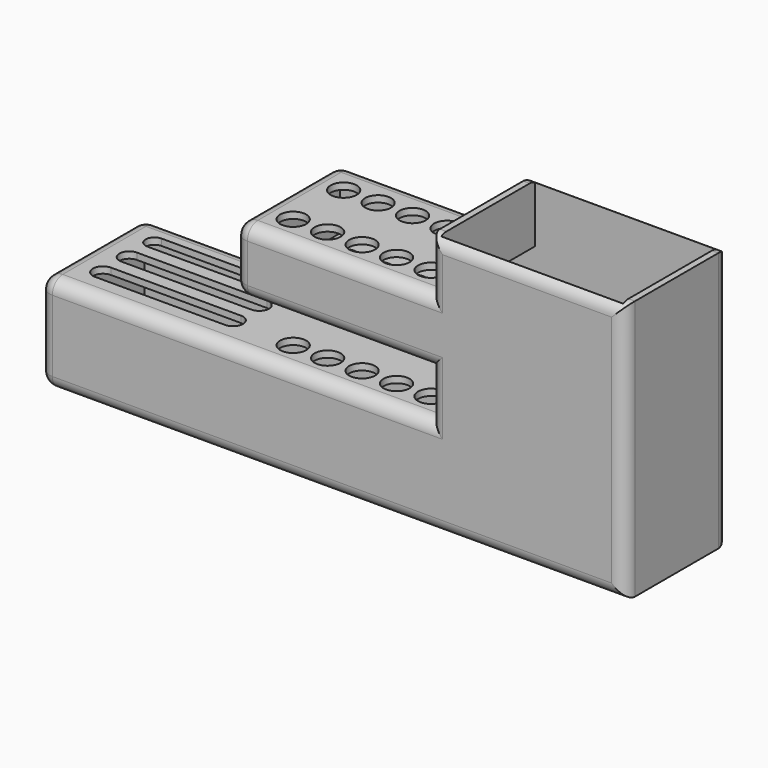
from build123d import *

# Parameters (mm, degrees)
F0_W          = 76.2
F0_H          = 25.4
F0_W_2        = 152.4
F0_H_2        = 38.1
F1_DEPTH      = 50.8
F2_T          = -2.54
F3_R          = 5.08
F4_DEPTH      = 76.2
F5_T1_DEPTH   = 101.6
F5_T3_DEPTH   = 32.8448284238
F5_T5_DEPTH   = 71.12
F5_T7_DEPTH   = 15.24
F5_T9_DEPTH   = 17.9551715762
F5_T11_DEPTH  = 147.32
F5_T13_DEPTH  = 27.94
F5_T15_DEPTH  = 236.22
F5_T17_DEPTH  = 127
F5_T19_DEPTH  = 40.64
F5_S23_W      = 5.08
F5_S23_H      = 5.08
F5_T24_DEPTH  = 5.08
F5_S29_W      = 5.08
F5_S29_H      = 5.08
F5_T30_DEPTH  = 5.08
F5_S35_W      = 5.08
F5_S35_H      = 5.08
F5_T36_DEPTH  = 5.08
F5_S41_W      = 5.08
F5_S41_H      = 5.08
F5_T42_DEPTH  = 5.08
F5_S47_W      = 5.08
F5_S47_H      = 5.08
F5_T48_DEPTH  = 5.08
F5_S53_W      = 5.08
F5_S53_H      = 5.08
F5_T54_DEPTH  = 5.08
F5_S59_W      = 5.08
F5_S59_H      = 5.08
F5_T60_DEPTH  = 5.08
F5_S65_W      = 5.08
F5_S65_H      = 5.08
F5_T66_DEPTH  = 5.08
F5_T73_DEPTH  = 45.5448284238
F5_T77_DEPTH  = 83.82
F5_T84_DEPTH  = 83.82
F5_T88_DEPTH  = 30.6551715762
F5_T95_DEPTH  = 30.6551715762
F5_T99_DEPTH  = 160.02
F5_T106_DEPTH = 45.5448284238
F5_T110_DEPTH = 83.82
F5_T117_DEPTH = 83.82
F5_T121_DEPTH = 30.6551715762
F5_T128_DEPTH = 30.6551715762
F5_T132_DEPTH = 160.02
F7_DEPTH      = 25.4


# Not quite as in the source:
# - a fillet or chamfer that OpenCascade refuses, or shapes differently, is made with other operations: its cross-section is extruded or revolved along the edge and cut away or added


with BuildPart() as f1:
    # F0 (on Front) → F1 (new body)
    with BuildSketch(Plane.XZ):
        Polygon((76.2, 45.5448284238), (0, 45.5448284238), (0, 25.4), (0, 0), (0, -17.9551715762), (0, -56.0551715762), (76.2, -56.0551715762), align=None)
        with Locations((-38.1, 12.7)):
            Rectangle(F0_W, F0_H)
        with Locations((-76.2, -37.0051715762)):
            Rectangle(F0_W_2, F0_H_2)
    extrude(amount=-F1_DEPTH)

    # F2
    f2_openings = [f1.faces().sort_by_distance(p)[0] for p in [
        (38.1, 25.4, 45.544828),
    ]]
    offset(amount=F2_T, openings=f2_openings, kind=Kind.INTERSECTION)

    # F3 (on face) → F4 (cut)
    with BuildSketch(Plane.XY.offset(25.4)):
        with Locations((-9.3213441366, 12.3962962994)):
            Circle(F3_R)
        with Locations((-9.3213441366, 37.0342962994)):
            Circle(F3_R)
        with Locations((-22.7833441366, 12.3962962994)):
            Circle(F3_R)
        with Locations((-22.7833441366, 37.0342962994)):
            Circle(F3_R)
        with Locations((-36.2453441366, 12.3962962994)):
            Circle(F3_R)
        with Locations((-36.2453441366, 37.0342962994)):
            Circle(F3_R)
        with Locations((-49.7073441366, 12.3962962994)):
            Circle(F3_R)
        with Locations((-49.7073441366, 37.0342962994)):
            Circle(F3_R)
        with Locations((-63.1693441366, 12.3962962994)):
            Circle(F3_R)
        with Locations((-63.1693441366, 37.0342962994)):
            Circle(F3_R)
    extrude(amount=-F4_DEPTH, mode=Mode.SUBTRACT)

    # F5: fillet of radius 5.08 on 24 edges, made by hand

    # F5_s2 → F5_t1 (cut)
    with BuildSketch(Plane.YZ.offset(-12.7)):
        with BuildLine():
            ThreePointArc((5.08, 45.5448284238), (1.4878975516, 44.0569308722), (0, 40.4648284238))
            Line((0, 40.4648284238), (0, 45.5448284238))
            Line((0, 45.5448284238), (5.08, 45.5448284238))
        make_face()
        with BuildLine():
            ThreePointArc((45.72, 45.5448284238), (49.3121024484, 44.0569308722), (50.8, 40.4648284238))
            Line((50.8, 40.4648284238), (50.8, 45.5448284238))
            Line((50.8, 45.5448284238), (45.72, 45.5448284238))
        make_face()
    extrude(amount=F5_T1_DEPTH, mode=Mode.SUBTRACT)

    # F5_s4 → F5_t3 (cut)
    with BuildSketch(Plane.XY.offset(25.4)):
        with BuildLine():
            ThreePointArc((0, 5.08), (1.4878975516, 1.4878975516), (5.08, 0))
            Line((5.08, 0), (0, 0))
            Line((0, 0), (0, 5.08))
        make_face()
        with BuildLine():
            ThreePointArc((0, 45.72), (1.4878975516, 49.3121024484), (5.08, 50.8))
            Line((5.08, 50.8), (0, 50.8))
            Line((0, 50.8), (0, 45.72))
        make_face()
    extrude(amount=F5_T3_DEPTH, mode=Mode.SUBTRACT)

    # F5_s6 → F5_t5 (cut)
    with BuildSketch(Plane.YZ.offset(-71.12)):
        with BuildLine():
            ThreePointArc((5.08, 25.4), (1.4878975516, 23.9121024484), (0, 20.32))
            Line((0, 20.32), (0, 25.4))
            Line((0, 25.4), (5.08, 25.4))
        make_face()
        with BuildLine():
            ThreePointArc((0, 5.08), (1.4878975516, 1.4878975516), (5.08, 0))
            Line((5.08, 0), (0, 0))
            Line((0, 0), (0, 5.08))
        make_face()
        with BuildLine():
            ThreePointArc((45.72, 25.4), (49.3121024484, 23.9121024484), (50.8, 20.32))
            Line((50.8, 20.32), (50.8, 25.4))
            Line((50.8, 25.4), (45.72, 25.4))
        make_face()
        with BuildLine():
            ThreePointArc((50.8, 5.08), (49.3121024484, 1.4878975516), (45.72, 0))
            Line((45.72, 0), (50.8, 0))
            Line((50.8, 0), (50.8, 5.08))
        make_face()
    extrude(amount=F5_T5_DEPTH, mode=Mode.SUBTRACT)

    # F5_s8 → F5_t7 (cut)
    with BuildSketch(Plane.XY.offset(5.08)):
        with BuildLine():
            ThreePointArc((-71.12, 0), (-74.7121024484, 1.4878975516), (-76.2, 5.08))
            Line((-76.2, 5.08), (-76.2, 0))
            Line((-76.2, 0), (-71.12, 0))
        make_face()
        with BuildLine():
            ThreePointArc((-71.12, 50.8), (-74.7121024484, 49.3121024484), (-76.2, 45.72))
            Line((-76.2, 45.72), (-76.2, 50.8))
            Line((-76.2, 50.8), (-71.12, 50.8))
        make_face()
    extrude(amount=F5_T7_DEPTH, mode=Mode.SUBTRACT)

    # F5_s10 → F5_t9 (cut)
    with BuildSketch(Plane.XY.offset(-17.9551715762)):
        with BuildLine():
            ThreePointArc((5.08, 0), (1.4878975516, 1.4878975516), (0, 5.08))
            Line((0, 5.08), (0, 0))
            Line((0, 0), (5.08, 0))
        make_face()
        with BuildLine():
            ThreePointArc((5.08, 50.8), (1.4878975516, 49.3121024484), (0, 45.72))
            Line((0, 45.72), (0, 50.8))
            Line((0, 50.8), (5.08, 50.8))
        make_face()
    extrude(amount=F5_T9_DEPTH, mode=Mode.SUBTRACT)

    # F5_s12 → F5_t11 (cut)
    with BuildSketch(Plane.YZ.offset(-147.32)):
        with BuildLine():
            ThreePointArc((0, -23.0351715762), (1.4878975516, -19.4430691278), (5.08, -17.9551715762))
            Line((5.08, -17.9551715762), (0, -17.9551715762))
            Line((0, -17.9551715762), (0, -23.0351715762))
        make_face()
        with BuildLine():
            ThreePointArc((50.8, -23.0351715762), (49.3121024484, -19.4430691278), (45.72, -17.9551715762))
            Line((45.72, -17.9551715762), (50.8, -17.9551715762))
            Line((50.8, -17.9551715762), (50.8, -23.0351715762))
        make_face()
    extrude(amount=F5_T11_DEPTH, mode=Mode.SUBTRACT)

    # F5_s14 → F5_t13 (cut)
    with BuildSketch(Plane.XY.offset(-50.9751715762)):
        with BuildLine():
            ThreePointArc((-147.32, 0), (-150.9121024484, 1.4878975516), (-152.4, 5.08))
            Line((-152.4, 5.08), (-152.4, 0))
            Line((-152.4, 0), (-147.32, 0))
        make_face()
        with BuildLine():
            ThreePointArc((-147.32, 50.8), (-150.9121024484, 49.3121024484), (-152.4, 45.72))
            Line((-152.4, 45.72), (-152.4, 50.8))
            Line((-152.4, 50.8), (-147.32, 50.8))
        make_face()
    extrude(amount=F5_T13_DEPTH, mode=Mode.SUBTRACT)

    # F5_s16 → F5_t15 (cut)
    with BuildSketch(Plane.YZ.offset(-147.32)):
        with BuildLine():
            ThreePointArc((0, -50.9751715762), (1.4878975516, -54.5672740246), (5.08, -56.0551715762))
            Line((5.08, -56.0551715762), (0, -56.0551715762))
            Line((0, -56.0551715762), (0, -50.9751715762))
        make_face()
        with BuildLine():
            ThreePointArc((50.8, -50.9751715762), (49.3121024484, -54.5672740246), (45.72, -56.0551715762))
            Line((45.72, -56.0551715762), (50.8, -56.0551715762))
            Line((50.8, -56.0551715762), (50.8, -50.9751715762))
        make_face()
    extrude(amount=F5_T15_DEPTH, mode=Mode.SUBTRACT)

    # F5_s18 → F5_t17 (cut)
    with BuildSketch(Plane.XY.offset(-68.7551715762)):
        with BuildLine():
            ThreePointArc((71.12, 0), (74.7121024484, 1.4878975516), (76.2, 5.08))
            Line((76.2, 5.08), (76.2, 0))
            Line((76.2, 0), (71.12, 0))
        make_face()
        with BuildLine():
            ThreePointArc((71.12, 50.8), (74.7121024484, 49.3121024484), (76.2, 45.72))
            Line((76.2, 45.72), (76.2, 50.8))
            Line((76.2, 50.8), (71.12, 50.8))
        make_face()
    extrude(amount=F5_T17_DEPTH, mode=Mode.SUBTRACT)

    # F5_s20 → F5_t19 (cut)
    with BuildSketch(Plane.XZ.offset(-45.72)):
        with BuildLine():
            ThreePointArc((-147.32, -17.9551715762), (-150.9121024484, -19.4430691278), (-152.4, -23.0351715762))
            Line((-152.4, -23.0351715762), (-152.4, -17.9551715762))
            Line((-152.4, -17.9551715762), (-147.32, -17.9551715762))
        make_face()
        with BuildLine():
            ThreePointArc((-152.4, -50.9751715762), (-150.9121024484, -54.5672740246), (-147.32, -56.0551715762))
            Line((-147.32, -56.0551715762), (-152.4, -56.0551715762))
            Line((-152.4, -56.0551715762), (-152.4, -50.9751715762))
        make_face()
        with BuildLine():
            ThreePointArc((-71.12, 25.4), (-74.7121024484, 23.9121024484), (-76.2, 20.32))
            Line((-76.2, 20.32), (-76.2, 25.4))
            Line((-76.2, 25.4), (-71.12, 25.4))
        make_face()
        with BuildLine():
            ThreePointArc((-76.2, 5.08), (-74.7121024484, 1.4878975516), (-71.12, 0))
            Line((-71.12, 0), (-76.2, 0))
            Line((-76.2, 0), (-76.2, 5.08))
        make_face()
    extrude(amount=F5_T19_DEPTH, mode=Mode.SUBTRACT)


with BuildPart() as f5_tool22:
    # F5_s23 → F5_t24 (new body)
    with BuildSketch(Plane.YZ.offset(-71.12)):
        with Locations((2.54, 22.86)):
            Rectangle(F5_S23_W, F5_S23_H)
    extrude(amount=-F5_T24_DEPTH)

    # F5_s25 → F5_t26 (revolve, cut)
    with BuildSketch(Plane(origin=(-71.12, 5.08, 20.32), x_dir=(0, 0.7071067812, -0.7071067812), z_dir=(0, 0.7071067812, 0.7071067812))):
        with BuildLine():
            ThreePointArc((0, -5.08), (5.08, 0), (0, 5.08))
            Line((0, 5.08), (0, -5.08))
        make_face()
    revolve(axis=Axis((-71.12, 5.08, 20.32), (-1, 0, 0)), mode=Mode.SUBTRACT)


with BuildPart() as f1_1:
    add(f1.part)

    # F5_t21: cut F5_tool22
    add(f5_tool22.part, mode=Mode.SUBTRACT)


with BuildPart() as f5_tool28:
    # F5_s29 → F5_t30 (new body)
    with BuildSketch(Plane.YZ.offset(-71.12)):
        with Locations((2.54, 2.54)):
            Rectangle(F5_S29_W, F5_S29_H)
    extrude(amount=-F5_T30_DEPTH)

    # F5_s31 → F5_t32 (revolve, cut)
    with BuildSketch(Plane(origin=(-71.12, 5.08, 5.08), x_dir=(0, 0.7071067812, 0.7071067812), z_dir=(0, -0.7071067812, 0.7071067812))):
        with BuildLine():
            ThreePointArc((0, -5.08), (5.08, 0), (0, 5.08))
            Line((0, 5.08), (0, -5.08))
        make_face()
    revolve(axis=Axis((-71.12, 5.08, 5.08), (-1, 0, 0)), mode=Mode.SUBTRACT)


with BuildPart() as f1_2:
    add(f1_1.part)

    # F5_t27: cut F5_tool28
    add(f5_tool28.part, mode=Mode.SUBTRACT)


with BuildPart() as f5_tool34:
    # F5_s35 → F5_t36 (new body)
    with BuildSketch(Plane.YZ.offset(-147.32)):
        with Locations((2.54, -20.4951715762)):
            Rectangle(F5_S35_W, F5_S35_H)
    extrude(amount=-F5_T36_DEPTH)

    # F5_s37 → F5_t38 (revolve, cut)
    with BuildSketch(Plane(origin=(-147.32, 5.08, -23.0351715762), x_dir=(0, 0.7071067812, -0.7071067812), z_dir=(0, 0.7071067812, 0.7071067812))):
        with BuildLine():
            ThreePointArc((0, -5.08), (5.08, 0), (0, 5.08))
            Line((0, 5.08), (0, -5.08))
        make_face()
    revolve(axis=Axis((-147.32, 5.08, -23.0351715762), (-1, 0, 0)), mode=Mode.SUBTRACT)


with BuildPart() as f1_3:
    add(f1_2.part)

    # F5_t33: cut F5_tool34
    add(f5_tool34.part, mode=Mode.SUBTRACT)


with BuildPart() as f5_tool40:
    # F5_s41 → F5_t42 (new body)
    with BuildSketch(Plane.YZ.offset(-147.32)):
        with Locations((2.54, -53.5151715762)):
            Rectangle(F5_S41_W, F5_S41_H)
    extrude(amount=-F5_T42_DEPTH)

    # F5_s43 → F5_t44 (revolve, cut)
    with BuildSketch(Plane(origin=(-147.32, 5.08, -50.9751715762), x_dir=(0, 0.7071067812, 0.7071067812), z_dir=(0, -0.7071067812, 0.7071067812))):
        with BuildLine():
            ThreePointArc((0, -5.08), (5.08, 0), (0, 5.08))
            Line((0, 5.08), (0, -5.08))
        make_face()
    revolve(axis=Axis((-147.32, 5.08, -50.9751715762), (-1, 0, 0)), mode=Mode.SUBTRACT)


with BuildPart() as f1_4:
    add(f1_3.part)

    # F5_t39: cut F5_tool40
    add(f5_tool40.part, mode=Mode.SUBTRACT)


with BuildPart() as f5_tool46:
    # F5_s47 → F5_t48 (new body)
    with BuildSketch(Plane.XY.offset(20.32)):
        with Locations((-73.66, 48.26)):
            Rectangle(F5_S47_W, F5_S47_H)
    extrude(amount=F5_T48_DEPTH)

    # F5_s49 → F5_t50 (revolve, cut)
    with BuildSketch(Plane(origin=(-71.12, 45.72, 20.32), x_dir=(0.7071067812, -0.7071067812, 0), z_dir=(-0.7071067812, -0.7071067812, 0))):
        with BuildLine():
            ThreePointArc((0, -5.08), (5.08, 0), (0, 5.08))
            Line((0, 5.08), (0, -5.08))
        make_face()
    revolve(axis=Axis((-71.12, 45.72, 20.32), (0, 0, 1)), mode=Mode.SUBTRACT)


with BuildPart() as f1_5:
    add(f1_4.part)

    # F5_t45: cut F5_tool46
    add(f5_tool46.part, mode=Mode.SUBTRACT)


with BuildPart() as f5_tool52:
    # F5_s53 → F5_t54 (new body)
    with BuildSketch(Plane.YZ.offset(-71.12)):
        with Locations((48.26, 2.54)):
            Rectangle(F5_S53_W, F5_S53_H)
    extrude(amount=-F5_T54_DEPTH)

    # F5_s55 → F5_t56 (revolve, cut)
    with BuildSketch(Plane(origin=(-71.12, 45.72, 5.08), x_dir=(0, -0.7071067812, 0.7071067812), z_dir=(0, -0.7071067812, -0.7071067812))):
        with BuildLine():
            ThreePointArc((0, -5.08), (5.08, 0), (0, 5.08))
            Line((0, 5.08), (0, -5.08))
        make_face()
    revolve(axis=Axis((-71.12, 45.72, 5.08), (-1, 0, 0)), mode=Mode.SUBTRACT)


with BuildPart() as f1_6:
    add(f1_5.part)

    # F5_t51: cut F5_tool52
    add(f5_tool52.part, mode=Mode.SUBTRACT)


with BuildPart() as f5_tool58:
    # F5_s59 → F5_t60 (new body)
    with BuildSketch(Plane.YZ.offset(-147.32)):
        with Locations((48.26, -20.4951715762)):
            Rectangle(F5_S59_W, F5_S59_H)
    extrude(amount=-F5_T60_DEPTH)

    # F5_s61 → F5_t62 (revolve, cut)
    with BuildSketch(Plane(origin=(-147.32, 45.72, -23.0351715762), x_dir=(0, -0.7071067812, -0.7071067812), z_dir=(0, 0.7071067812, -0.7071067812))):
        with BuildLine():
            ThreePointArc((0, -5.08), (5.08, 0), (0, 5.08))
            Line((0, 5.08), (0, -5.08))
        make_face()
    revolve(axis=Axis((-147.32, 45.72, -23.0351715762), (-1, 0, 0)), mode=Mode.SUBTRACT)


with BuildPart() as f1_7:
    add(f1_6.part)

    # F5_t57: cut F5_tool58
    add(f5_tool58.part, mode=Mode.SUBTRACT)


with BuildPart() as f5_tool64:
    # F5_s65 → F5_t66 (new body)
    with BuildSketch(Plane.YZ.offset(-147.32)):
        with Locations((48.26, -53.5151715762)):
            Rectangle(F5_S65_W, F5_S65_H)
    extrude(amount=-F5_T66_DEPTH)

    # F5_s67 → F5_t68 (revolve, cut)
    with BuildSketch(Plane(origin=(-147.32, 45.72, -50.9751715762), x_dir=(0, -0.7071067812, 0.7071067812), z_dir=(0, -0.7071067812, -0.7071067812))):
        with BuildLine():
            ThreePointArc((0, -5.08), (5.08, 0), (0, 5.08))
            Line((0, 5.08), (0, -5.08))
        make_face()
    revolve(axis=Axis((-147.32, 45.72, -50.9751715762), (-1, 0, 0)), mode=Mode.SUBTRACT)


with BuildPart() as f1_8:
    add(f1_7.part)

    # F5_t63: cut F5_tool64
    add(f5_tool64.part, mode=Mode.SUBTRACT)


with BuildPart() as f5_tool71:
    # F5_s72 → F5_t73 (new body)
    with BuildSketch(Plane.XY.offset(58.2448284238)):
        with BuildLine():
            ThreePointArc((0, 5.08), (1.4878975516, 1.4878975516), (5.08, 0))
            Line((5.08, 0), (0, 0))
            Line((0, 0), (0, 5.08))
        make_face()
    extrude(amount=-F5_T73_DEPTH)

    split(bisect_by=Plane.XY.offset(25.4), keep=Keep.BOTTOM)


with BuildPart() as f5_tool75:
    # F5_s76 → F5_t77 (new body)
    with BuildSketch(Plane.YZ.offset(12.7)):
        with BuildLine():
            ThreePointArc((5.08, 25.4), (1.4878975516, 23.9121024484), (0, 20.32))
            Line((0, 20.32), (0, 25.4))
            Line((0, 25.4), (5.08, 25.4))
        make_face()
    extrude(amount=-F5_T77_DEPTH)

    split(bisect_by=Plane.YZ, keep=Keep.TOP)


with BuildPart() as f5_tool71_1:
    add(f5_tool71.part)

    # F5_t79: intersect F5_tool75
    add(f5_tool75.part, mode=Mode.INTERSECT)


with BuildPart() as f1_9:
    add(f1_8.part)

    # F5_t69: cut F5_tool71
    add(f5_tool71_1.part, mode=Mode.SUBTRACT)


with BuildPart() as f5_tool82:
    # F5_s83 → F5_t84 (new body)
    with BuildSketch(Plane.YZ.offset(-71.12)):
        with BuildLine():
            ThreePointArc((0, 5.08), (1.4878975516, 1.4878975516), (5.08, 0))
            Line((5.08, 0), (0, 0))
            Line((0, 0), (0, 5.08))
        make_face()
    extrude(amount=F5_T84_DEPTH)

    split(bisect_by=Plane.YZ, keep=Keep.TOP)


with BuildPart() as f5_tool86:
    # F5_s87 → F5_t88 (new body)
    with BuildSketch(Plane.XY.offset(12.7)):
        with BuildLine():
            ThreePointArc((5.08, 0), (1.4878975516, 1.4878975516), (0, 5.08))
            Line((0, 5.08), (0, 0))
            Line((0, 0), (5.08, 0))
        make_face()
    extrude(amount=-F5_T88_DEPTH)

    split(bisect_by=Plane.XY, keep=Keep.TOP)


with BuildPart() as f5_tool82_1:
    add(f5_tool82.part)

    # F5_t90: intersect F5_tool86
    add(f5_tool86.part, mode=Mode.INTERSECT)


with BuildPart() as f1_10:
    add(f1_9.part)

    # F5_t80: cut F5_tool82
    add(f5_tool82_1.part, mode=Mode.SUBTRACT)


with BuildPart() as f5_tool93:
    # F5_s94 → F5_t95 (new body)
    with BuildSketch(Plane.XY):
        with BuildLine():
            ThreePointArc((5.08, 0), (1.4878975516, 1.4878975516), (0, 5.08))
            Line((0, 5.08), (0, 0))
            Line((0, 0), (5.08, 0))
        make_face()
    extrude(amount=-F5_T95_DEPTH)

    split(bisect_by=Plane.XY.offset(-17.9551715762), keep=Keep.BOTTOM)


with BuildPart() as f5_tool97:
    # F5_s98 → F5_t99 (new body)
    with BuildSketch(Plane.YZ.offset(12.7)):
        with BuildLine():
            ThreePointArc((0, -23.0351715762), (1.4878975516, -19.4430691278), (5.08, -17.9551715762))
            Line((5.08, -17.9551715762), (0, -17.9551715762))
            Line((0, -17.9551715762), (0, -23.0351715762))
        make_face()
    extrude(amount=-F5_T99_DEPTH)

    split(bisect_by=Plane.YZ, keep=Keep.TOP)


with BuildPart() as f5_tool93_1:
    add(f5_tool93.part)

    # F5_t101: intersect F5_tool97
    add(f5_tool97.part, mode=Mode.INTERSECT)


with BuildPart() as f1_11:
    add(f1_10.part)

    # F5_t91: cut F5_tool93
    add(f5_tool93_1.part, mode=Mode.SUBTRACT)


with BuildPart() as f5_tool104:
    # F5_s105 → F5_t106 (new body)
    with BuildSketch(Plane.XY.offset(58.2448284238)):
        with BuildLine():
            ThreePointArc((0, 45.72), (1.4878975516, 49.3121024484), (5.08, 50.8))
            Line((5.08, 50.8), (0, 50.8))
            Line((0, 50.8), (0, 45.72))
        make_face()
    extrude(amount=-F5_T106_DEPTH)

    split(bisect_by=Plane.XY.offset(25.4), keep=Keep.BOTTOM)


with BuildPart() as f5_tool108:
    # F5_s109 → F5_t110 (new body)
    with BuildSketch(Plane.YZ.offset(12.7)):
        with BuildLine():
            ThreePointArc((45.72, 25.4), (49.3121024484, 23.9121024484), (50.8, 20.32))
            Line((50.8, 20.32), (50.8, 25.4))
            Line((50.8, 25.4), (45.72, 25.4))
        make_face()
    extrude(amount=-F5_T110_DEPTH)

    split(bisect_by=Plane.YZ, keep=Keep.TOP)


with BuildPart() as f5_tool104_1:
    add(f5_tool104.part)

    # F5_t112: intersect F5_tool108
    add(f5_tool108.part, mode=Mode.INTERSECT)


with BuildPart() as f1_12:
    add(f1_11.part)

    # F5_t102: cut F5_tool104
    add(f5_tool104_1.part, mode=Mode.SUBTRACT)


with BuildPart() as f5_tool115:
    # F5_s116 → F5_t117 (new body)
    with BuildSketch(Plane.YZ.offset(-71.12)):
        with BuildLine():
            ThreePointArc((50.8, 5.08), (49.3121024484, 1.4878975516), (45.72, 0))
            Line((45.72, 0), (50.8, 0))
            Line((50.8, 0), (50.8, 5.08))
        make_face()
    extrude(amount=F5_T117_DEPTH)

    split(bisect_by=Plane.YZ, keep=Keep.TOP)


with BuildPart() as f5_tool119:
    # F5_s120 → F5_t121 (new body)
    with BuildSketch(Plane.XY.offset(12.7)):
        with BuildLine():
            ThreePointArc((5.08, 50.8), (1.4878975516, 49.3121024484), (0, 45.72))
            Line((0, 45.72), (0, 50.8))
            Line((0, 50.8), (5.08, 50.8))
        make_face()
    extrude(amount=-F5_T121_DEPTH)

    split(bisect_by=Plane.XY, keep=Keep.TOP)


with BuildPart() as f5_tool115_1:
    add(f5_tool115.part)

    # F5_t123: intersect F5_tool119
    add(f5_tool119.part, mode=Mode.INTERSECT)


with BuildPart() as f1_13:
    add(f1_12.part)

    # F5_t113: cut F5_tool115
    add(f5_tool115_1.part, mode=Mode.SUBTRACT)


with BuildPart() as f5_tool126:
    # F5_s127 → F5_t128 (new body)
    with BuildSketch(Plane.XY):
        with BuildLine():
            ThreePointArc((5.08, 50.8), (1.4878975516, 49.3121024484), (0, 45.72))
            Line((0, 45.72), (0, 50.8))
            Line((0, 50.8), (5.08, 50.8))
        make_face()
    extrude(amount=-F5_T128_DEPTH)

    split(bisect_by=Plane.XY.offset(-17.9551715762), keep=Keep.BOTTOM)


with BuildPart() as f5_tool130:
    # F5_s131 → F5_t132 (new body)
    with BuildSketch(Plane.YZ.offset(12.7)):
        with BuildLine():
            ThreePointArc((50.8, -23.0351715762), (49.3121024484, -19.4430691278), (45.72, -17.9551715762))
            Line((45.72, -17.9551715762), (50.8, -17.9551715762))
            Line((50.8, -17.9551715762), (50.8, -23.0351715762))
        make_face()
    extrude(amount=-F5_T132_DEPTH)

    split(bisect_by=Plane.YZ, keep=Keep.TOP)


with BuildPart() as f5_tool126_1:
    add(f5_tool126.part)

    # F5_t134: intersect F5_tool130
    add(f5_tool130.part, mode=Mode.INTERSECT)


with BuildPart() as f1_14:
    add(f1_13.part)

    # F5_t124: cut F5_tool126
    add(f5_tool126_1.part, mode=Mode.SUBTRACT)

    # F6 (on face) → F7 (cut)
    with BuildSketch(Plane.XY.offset(-17.9551715762)):
        with BuildLine():
            ThreePointArc((-138.6253818214, 17.7800003439), (-142.5330744401, 13.8723077253), (-138.6253818214, 9.9646151066))
            Line((-138.6253818214, 9.9646151066), (-87.8253818214, 9.9646151066))
            ThreePointArc((-87.8253818214, 9.9646151066), (-83.9176892027, 13.8723077253), (-87.8253818214, 17.7800003439))
            Line((-87.8253818214, 17.7800003439), (-138.6253818214, 17.7800003439))
        make_face()
        with BuildLine():
            ThreePointArc((-138.6253818214, 30.4800003439), (-142.4353818214, 26.6700003439), (-138.6253818214, 22.8600003439))
            Line((-138.6253818214, 22.8600003439), (-87.8253818214, 22.8600003439))
            ThreePointArc((-87.8253818214, 22.8600003439), (-84.0153818214, 26.6700003439), (-87.8253818214, 30.4800003439))
            Line((-87.8253818214, 30.4800003439), (-138.6253818214, 30.4800003439))
        make_face()
        with BuildLine():
            ThreePointArc((-138.6253818214, 42.3984639347), (-142.0446136168, 38.9792321393), (-138.6253818214, 35.5600003439))
            Line((-138.6253818214, 35.5600003439), (-87.8253818214, 35.5600003439))
            ThreePointArc((-87.8253818214, 35.5600003439), (-84.406150026, 38.9792321393), (-87.8253818214, 42.3984639347))
            Line((-87.8253818214, 42.3984639347), (-138.6253818214, 42.3984639347))
        make_face()
    extrude(amount=-F7_DEPTH, mode=Mode.SUBTRACT)


solid = f1_14.part
